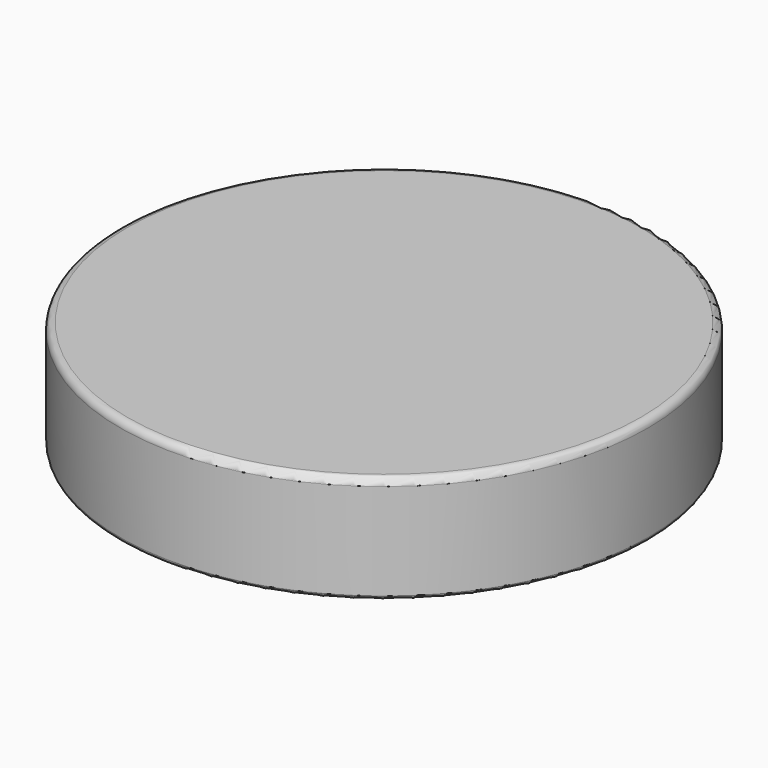
from build123d import *

# Parameters (mm, degrees)
F0_R     = 37
F0_R_2   = 36
F1_DEPTH = 15
F2_R     = 36.9218427358
F3_DEPTH = 2
F4_R     = 1
F5_R     = 0.49999


# Not quite as in the source:
# - a fillet or chamfer is up to 0.001 mm smaller than in the source, because OpenCascade refuses the exact size


with BuildPart() as f1:
    # F0 (on Top) → F1 (new body)
    with BuildSketch(Plane.XY):
        Circle(F0_R)
        Circle(F0_R_2, mode=Mode.SUBTRACT)
    extrude(amount=F1_DEPTH)

    # F2 (on face) → F3 (join)
    with BuildSketch(Plane.XY.offset(15)):
        Circle(F2_R)
    extrude(amount=-F3_DEPTH)

    # F4
    f4_edges = [f1.edges().sort_by_distance(p)[0] for p in [
        (-37, 0, 15),
    ]]
    fillet(f4_edges, radius=F4_R)

    # F5 (radius 0.5 in the source; OpenCascade refuses exactly that, so slightly less here)
    f5_edges = [f1.edges().sort_by_distance(p)[0] for p in [
        (-37, 0, 0),
        (-36, 0, 0),
    ]]
    fillet(f5_edges, radius=F5_R)


solid = f1.part
